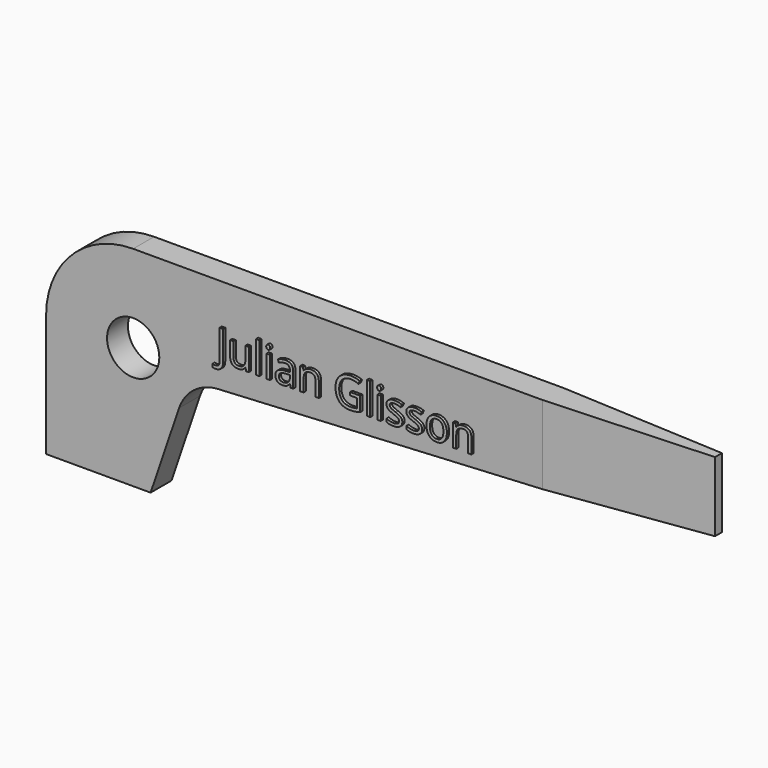
from build123d import *

# Parameters (mm, degrees)
F1_DEPTH     = 2.38125
F2_R         = 2.38125
F3_DEPTH     = 2.38225
F5_DEPTH     = 25.4
F6_TEXT_SIZE = 3.794677956
F7_DEPTH     = 0.254


# Not quite as in the source:
# - Text() gives the source's letters only with a copy of the font that has no kerning and outlines rounded to 1/6400 em; it was checked with that copy


with BuildPart() as f1:
    # F0 (on Front) → F1 (new body)
    with BuildSketch(Plane.XZ):
        with BuildLine():
            Line((60.325, 19.05), (7.9375, 19.05))
            ThreePointArc((7.9375, 19.05), (2.3248399243, 16.7251600757), (0, 11.1125))
            Line((0, 11.1125), (0, 0))
            Line((0, 0), (9.525, 0))
            Line((9.525, 0), (12.1173647876, 7.6271664624))
            ThreePointArc((12.1173647876, 7.6271664624), (13.4786145605, 9.5135918491), (15.6631963617, 10.3130942181))
            Line((15.6631963617, 10.3130942181), (60.325, 12.7))
            Line((60.325, 12.7), (60.325, 19.05))
        make_face()
    extrude(amount=F1_DEPTH)

    # F2 (on face) → F3 (cut, through all)
    with BuildSketch(Plane.XZ.offset(2.38125)):
        with Locations((7.9375, 11.1125)):
            Circle(F2_R)
    extrude(amount=-F3_DEPTH, mode=Mode.SUBTRACT)

    # F4 (on face) → F5 (cut)
    with BuildSketch(Plane.XY.offset(19.05)):
        Polygon((60.325, -2.38125), (60.325, -1.5875), (45.24375, -2.38125), align=None)
        Polygon((60.325, 0), (45.24375, 0), (60.325, -0.79375), align=None)
    extrude(amount=-F5_DEPTH, mode=Mode.SUBTRACT)

    # F6 (on face) → F7 (join)
    with BuildSketch(Plane.XZ.offset(2.38125)):
        with Locations((15.6631963617, 12.7398306504)):
            Text('Julian Glisson', F6_TEXT_SIZE, font='Open Sans', text_align=(TextAlign.LEFT, TextAlign.BOTTOM))
    extrude(amount=F7_DEPTH)


solid = f1.part
